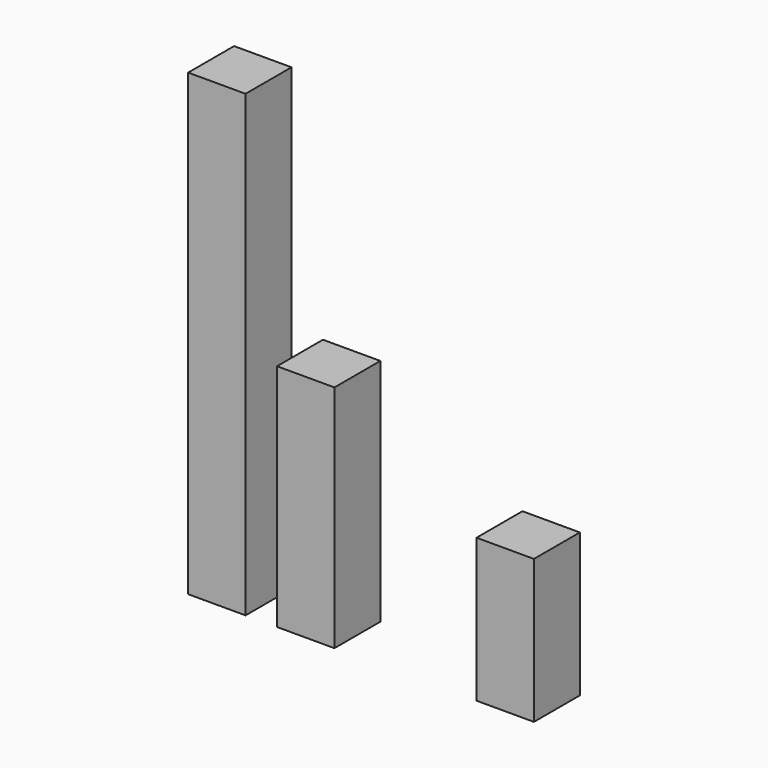
from build123d import *

# Parameters (mm, degrees)
F0_W     = 50
F0_H     = 400
F1_DEPTH = 50
F0_H_2   = 200
F0_H_3   = 125


# Not quite as in the source:
# - a feature names something its author has since deleted; it is built from what else it names


with BuildPart() as f1:
    # F0 (on Front) → F1 (new body)
    with BuildSketch(Plane.XZ):
        with Locations((-27.8219481464, 135.4479238391)):
            Rectangle(F0_W, F0_H)
    extrude(amount=F1_DEPTH)


with BuildPart() as f1b:
    # F0 (on Front) → F1, piece 2 (new body)
    with BuildSketch(Plane.XZ):
        with Locations((49.590652436, 35.4479238391)):
            Rectangle(F0_W, F0_H_2)
    extrude(amount=F1_DEPTH)


with BuildPart() as f1c:
    # F0 (on Front) → F1, piece 3 (new body)
    with BuildSketch(Plane.XZ):
        with Locations((223.378162575, -2.0520761609)):
            Rectangle(F0_W, F0_H_3)
    extrude(amount=F1_DEPTH)


solid = Compound([f1.part, f1b.part, f1c.part])
